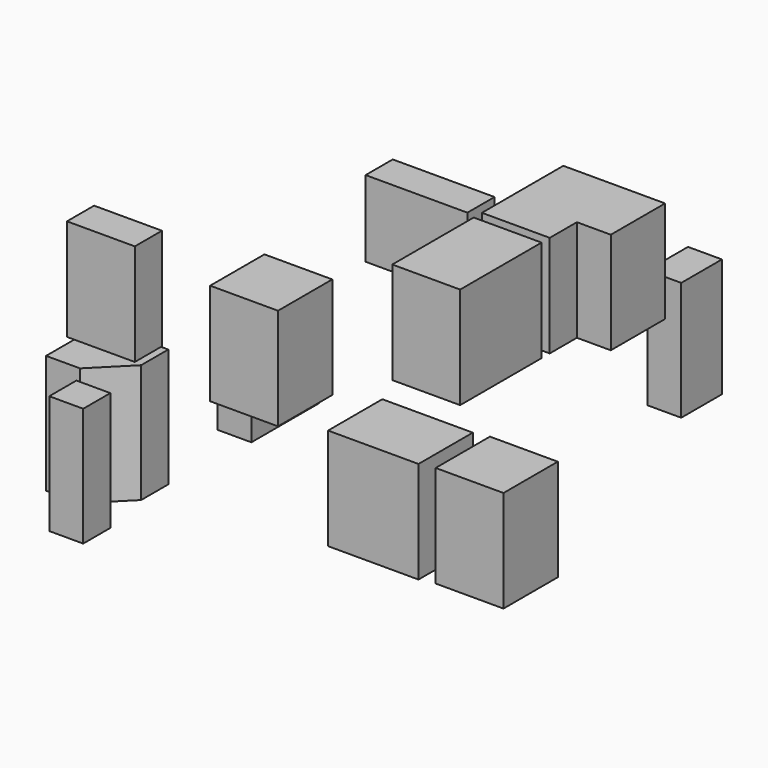
from build123d import *

# Parameters (mm, degrees)
F0_W      = 609.6
F0_H      = 914.4
F1_DEPTH  = 914.4
F3_DEPTH  = 914.4
F4_W      = 609.6
F4_H      = 609.6
F5_DEPTH  = 914.4
F6_W      = 812.8
F6_H      = 609.6
F7_DEPTH  = 914.4
F8_W      = 609.6
F8_H      = 609.6
F9_DEPTH  = 914.4
F10_W     = 609.6
F10_H     = 304.8
F11_DEPTH = 914.4
F13_DEPTH = 1066.8
F14_W     = 304.8
F14_H     = 304.8
F15_DEPTH = 1066.8
F16_W     = 304.8
F16_H     = 762
F17_DEPTH = 762
F18_W     = 914.4
F18_H     = 304.8
F19_DEPTH = 685.8
F20_W     = 304.8
F20_H     = 457.2
F21_DEPTH = 1066.8


# Not quite as in the source:
# - a feature names something its author has since deleted; it is built from what else it names


with BuildPart() as f1:
    # F0 (on Top) → F1 (new body)
    with BuildSketch(Plane.XY):
        with Locations((-50.6302136928, 46.2002533887)):
            Rectangle(F0_W, F0_H)
    extrude(amount=F1_DEPTH)


with BuildPart() as f3:
    # F2 (on face) → F3 (new body)
    with BuildSketch(Plane(origin=(0, 0, 0), x_dir=(1, 0, 0), z_dir=(0, 0, -1))):
        Polygon((254.1697863072, -900.2123884309), (254.1697863072, -595.4123884309), (-355.4302136928, -595.4123884309), (-355.4302136928, -1509.8123884309), (558.9697863072, -1509.8123884309), (558.9697863072, -900.2123884309), align=None)
    extrude(amount=-F3_DEPTH)


with BuildPart() as f5:
    # F4 (on face) → F5 (new body)
    with BuildSketch(Plane(origin=(0, 0, 0), x_dir=(1, 0, 0), z_dir=(0, 0, -1))):
        with Locations((1020.5837786198, 958.2468374996)):
            Rectangle(F4_W, F4_H)
    extrude(amount=F5_DEPTH)


with BuildPart() as f7:
    # F6 (on face) → F7 (new body)
    with BuildSketch(Plane(origin=(0, 0, 0), x_dir=(1, 0, 0), z_dir=(0, 0, -1))):
        with Locations((177.7652353048, 986.2984619199)):
            Rectangle(F6_W, F6_H)
    extrude(amount=F7_DEPTH)


with BuildPart() as f9:
    # F8 (on face) → F9 (new body)
    with BuildSketch(Plane.XY):
        with Locations((-847.6822674274, -1155.6124973011)):
            Rectangle(F8_W, F8_H)
    extrude(amount=F9_DEPTH)


with BuildPart() as f11:
    # F10 (on face) → F11 (new body)
    with BuildSketch(Plane.XY.offset(914.4)):
        with Locations((-1145.7255238362, -2543.5986241634)):
            Rectangle(F10_W, F10_H)
    extrude(amount=F11_DEPTH)


with BuildPart() as f13:
    # F12 (on face) → F13 (new body)
    with BuildSketch(Plane(origin=(0, 0, 0), x_dir=(1, 0, 0), z_dir=(0, 0, -1))):
        Polygon((-2482.6113088184, 1029.8828289854), (-1873.0113088184, 1029.8828289854), (-1873.0113088184, 1334.6828289854), (-2177.8113088184, 1640.5393312868), (-2482.6113088184, 1640.5393312868), align=None)
    extrude(amount=F13_DEPTH)


with BuildPart() as f15:
    # F14 (on face) → F15 (new body)
    with BuildSketch(Plane(origin=(0, 0, 0), x_dir=(1, 0, 0), z_dir=(0, 0, -1))):
        with Locations((-1929.4477705223, 1953.2716274261)):
            Rectangle(F14_W, F14_H)
    extrude(amount=F15_DEPTH)


with BuildPart() as f17:
    # F16 (on face) → F17 (new body)
    with BuildSketch(Plane(origin=(0, 0, 0), x_dir=(1, 0, 0), z_dir=(0, 0, -1))):
        with Locations((-1603.5444736481, 243.1021227015)):
            Rectangle(F16_W, F16_H)
    extrude(amount=F17_DEPTH)


with BuildPart() as f19:
    # F18 (on face) → F19 (new body)
    with BuildSketch(Plane(origin=(0, 0, 0), x_dir=(1, 0, 0), z_dir=(0, 0, -1))):
        with Locations((-1990.6274676323, -2057.3001701469)):
            Rectangle(F18_W, F18_H)
    extrude(amount=F19_DEPTH)


with BuildPart() as f21:
    # F20 (on face) → F21 (new body)
    with BuildSketch(Plane(origin=(0, 0, 0), x_dir=(1, 0, 0), z_dir=(0, 0, -1))):
        with Locations((152.4, -2237.3750410851)):
            Rectangle(F20_W, F20_H)
    extrude(amount=F21_DEPTH)


solid = Compound([f1.part, f3.part, f5.part, f7.part, f9.part, f11.part, f13.part, f15.part, f17.part, f19.part, f21.part])
